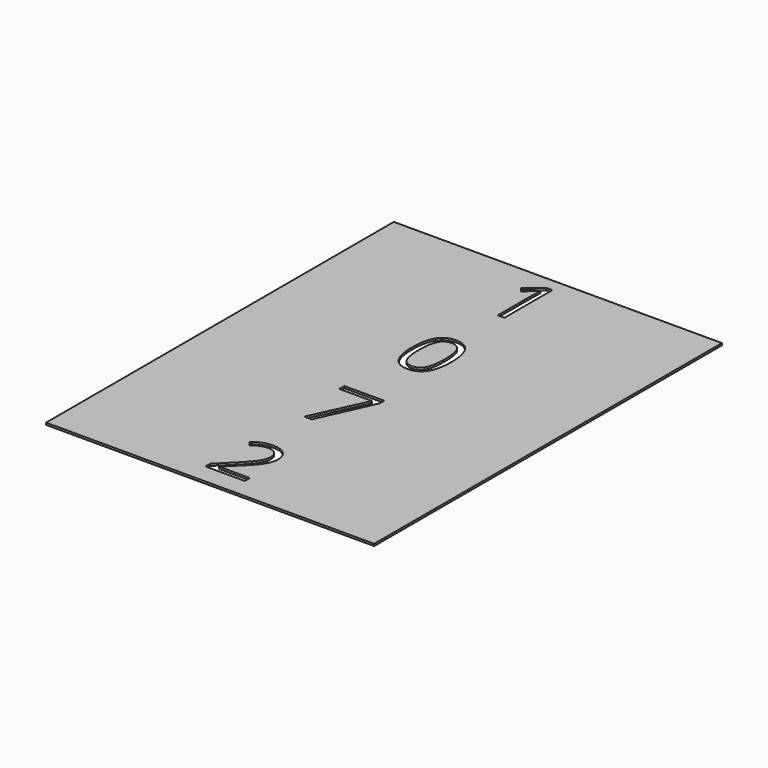
from build123d import *

# Parameters (mm, degrees)
F0_W     = 508
F0_H     = 673.1
F1_DEPTH = 3.175


# Not quite as in the source:
# - a feature names something its author has since deleted; it is built from what else it names


with BuildPart() as f1:
    # F0 (on Top) → F1 (new body)
    with BuildSketch(Plane.XY):
        with Locations((254, -336.55)):
            Rectangle(F0_W, F0_H)
        with BuildLine():
            Line((283.1734824281, -632.5249201278), (283.1734824281, -642.2832268371))
            Line((283.1734824281, -642.2832268371), (222.25, -642.2832268371))
            Line((222.25, -642.2832268371), (222.25, -633.2146964856))
            Line((222.25, -633.2146964856), (246.6559105431, -608.6870607029))
            add(Edge.make_bspline(
                [(246.6559105431, -608.6870607029), (257.814057508, -597.3869009585), (261.3643769968, -592.5686102236)],
                knots=[0, 0, 0, 1, 1, 1], degree=2))
            add(Edge.make_bspline(
                [(261.3643769968, -592.5686102236), (264.9146964856, -587.7503194888), (266.68985623, -583.1856230032)],
                knots=[0, 0, 0, 1, 1, 1], degree=2))
            add(Edge.make_bspline(
                [(266.68985623, -583.1856230032), (268.4650159744, -578.6209265176), (268.4650159744, -573.3664536741)],
                knots=[0, 0, 0, 1, 1, 1], degree=2))
            add(Edge.make_bspline(
                [(268.4650159744, -573.3664536741), (268.4650159744, -565.9412140575), (263.9611821086, -561.5996805112)],
                knots=[0, 0, 0, 1, 1, 1], degree=2))
            add(Edge.make_bspline(
                [(263.9611821086, -561.5996805112), (259.4573482428, -557.2581469649), (251.464057508, -557.2581469649)],
                knots=[0, 0, 0, 1, 1, 1], degree=2))
            add(Edge.make_bspline(
                [(251.464057508, -557.2581469649), (245.7023961661, -557.2581469649), (240.5290734824, -559.1651757189)],
                knots=[0, 0, 0, 1, 1, 1], degree=2))
            add(Edge.make_bspline(
                [(240.5290734824, -559.1651757189), (235.3557507987, -561.0722044728), (229.0260383387, -566.0832268371)],
                knots=[0, 0, 0, 1, 1, 1], degree=2))
            Line((229.0260383387, -566.0832268371), (223.4469648562, -558.9217252396))
            add(Edge.make_bspline(
                [(223.4469648562, -558.9217252396), (236.2484025559, -548.2707667732), (251.3423322684, -548.2707667732)],
                knots=[0, 0, 0, 1, 1, 1], degree=2))
            add(Edge.make_bspline(
                [(251.3423322684, -548.2707667732), (264.4075079872, -548.2707667732), (271.8226038339, -554.9555111821)],
                knots=[0, 0, 0, 1, 1, 1], degree=2))
            add(Edge.make_bspline(
                [(271.8226038339, -554.9555111821), (279.2376996805, -561.6402555911), (279.2376996805, -572.9201277955)],
                knots=[0, 0, 0, 1, 1, 1], degree=2))
            add(Edge.make_bspline(
                [(279.2376996805, -572.9201277955), (279.2376996805, -581.7452076677), (274.2875399361, -590.3674121406)],
                knots=[0, 0, 0, 1, 1, 1], degree=2))
            add(Edge.make_bspline(
                [(274.2875399361, -590.3674121406), (269.3373801917, -598.9896166134), (255.7853035144, -612.1765175719)],
                knots=[0, 0, 0, 1, 1, 1], degree=2))
            Line((255.7853035144, -612.1765175719), (235.4977635783, -632.0177316294))
            Line((235.4977635783, -632.0177316294), (235.4977635783, -632.5249201278))
            Line((235.4977635783, -632.5249201278), (283.1734824281, -632.5249201278))
        make_face(mode=Mode.SUBTRACT)
        Polygon((245.6415335463, -465.7004792332), (233.9761980831, -465.7004792332), (272.3805111821, -382.7041533546), (221.8645367412, -382.7041533546), (221.8645367412, -373.0067092652), (283.538658147, -373.0067092652), (283.538658147, -381.4463258786), align=None, mode=Mode.SUBTRACT)
        with BuildLine():
            add(Edge.make_bspline(
                [(275.8496805112, -207.2067891374), (283.6806709265, -219.4503194888), (283.6806709265, -242.6389776358)],
                knots=[0, 0, 0, 1, 1, 1], degree=2))
            add(Edge.make_bspline(
                [(283.6806709265, -242.6389776358), (283.6806709265, -266.6797124601), (276.1032747604, -278.5377795527)],
                knots=[0, 0, 0, 1, 1, 1], degree=2))
            add(Edge.make_bspline(
                [(276.1032747604, -278.5377795527), (268.5258785942, -290.3958466454), (252.9247603834, -290.3958466454)],
                knots=[0, 0, 0, 1, 1, 1], degree=2))
            add(Edge.make_bspline(
                [(252.9247603834, -290.3958466454), (237.9728434505, -290.3958466454), (230.172284345, -278.2537539936)],
                knots=[0, 0, 0, 1, 1, 1], degree=2))
            add(Edge.make_bspline(
                [(230.172284345, -278.2537539936), (222.3717252396, -266.1116613419), (222.3717252396, -242.6389776358)],
                knots=[0, 0, 0, 1, 1, 1], degree=2))
            add(Edge.make_bspline(
                [(222.3717252396, -242.6389776358), (222.3717252396, -218.435942492), (229.9186900958, -206.699600639)],
                knots=[0, 0, 0, 1, 1, 1], degree=2))
            add(Edge.make_bspline(
                [(229.9186900958, -206.699600639), (237.4656549521, -194.9632587859), (252.9247603834, -194.9632587859)],
                knots=[0, 0, 0, 1, 1, 1], degree=2))
            add(Edge.make_bspline(
                [(252.9247603834, -194.9632587859), (268.0186900958, -194.9632587859), (275.8496805112, -207.2067891374)],
                knots=[0, 0, 0, 1, 1, 1], degree=2))
        make_face(mode=Mode.SUBTRACT)
        with BuildLine():
            Line((261.2223642173, -19.8412140575), (261.2223642173, -112.5349840256))
            Line((261.2223642173, -112.5349840256), (250.9568690096, -112.5349840256))
            Line((250.9568690096, -112.5349840256), (250.9568690096, -46.4787539936))
            add(Edge.make_bspline(
                [(250.9568690096, -46.4787539936), (250.9568690096, -38.2217252396), (251.464057508, -30.8776357827)],
                knots=[0, 0, 0, 1, 1, 1], degree=2))
            add(Edge.make_bspline(
                [(251.464057508, -30.8776357827), (250.1453674121, -32.2166134185), (248.4919329073, -33.667172524)],
                knots=[0, 0, 0, 1, 1, 1], degree=2))
            add(Edge.make_bspline(
                [(248.4919329073, -33.667172524), (246.8384984026, -35.1177316294), (233.4081469649, -46.032428115)],
                knots=[0, 0, 0, 1, 1, 1], degree=2))
            Line((233.4081469649, -46.032428115), (227.8290734824, -38.8100638978))
            Line((227.8290734824, -38.8100638978), (252.3567092652, -19.8412140575))
            Line((252.3567092652, -19.8412140575), (261.2223642173, -19.8412140575))
        make_face(mode=Mode.SUBTRACT)
    extrude(amount=F1_DEPTH)


with BuildPart() as f1b:
    # F0 (on Top) → F1, piece 2 (new body)
    with BuildSketch(Plane.XY):
        with BuildLine():
            add(Edge.make_bspline(
                [(237.7801118211, -213.2524760383), (233.0226837061, -222.4123003195), (233.0226837061, -242.6389776358)],
                knots=[0, 0, 0, 1, 1, 1], degree=2))
            add(Edge.make_bspline(
                [(233.0226837061, -242.6389776358), (233.0226837061, -262.8656549521), (237.7801118211, -272.096485623)],
                knots=[0, 0, 0, 1, 1, 1], degree=2))
            add(Edge.make_bspline(
                [(237.7801118211, -272.096485623), (242.5375399361, -281.3273162939), (252.9247603834, -281.3273162939)],
                knots=[0, 0, 0, 1, 1, 1], degree=2))
            add(Edge.make_bspline(
                [(252.9247603834, -281.3273162939), (263.4539936102, -281.3273162939), (268.1708466454, -271.9747603834)],
                knots=[0, 0, 0, 1, 1, 1], degree=2))
            add(Edge.make_bspline(
                [(268.1708466454, -271.9747603834), (272.8876996805, -262.6222044728), (272.8876996805, -242.6389776358)],
                knots=[0, 0, 0, 1, 1, 1], degree=2))
            add(Edge.make_bspline(
                [(272.8876996805, -242.6389776358), (272.8876996805, -222.6760383387), (268.1708466454, -213.3843450479)],
                knots=[0, 0, 0, 1, 1, 1], degree=2))
            add(Edge.make_bspline(
                [(268.1708466454, -213.3843450479), (263.4539936102, -204.0926517572), (252.9247603834, -204.0926517572)],
                knots=[0, 0, 0, 1, 1, 1], degree=2))
            add(Edge.make_bspline(
                [(252.9247603834, -204.0926517572), (242.5375399361, -204.0926517572), (237.7801118211, -213.2524760383)],
                knots=[0, 0, 0, 1, 1, 1], degree=2))
        make_face()
    extrude(amount=F1_DEPTH)


solid = Compound([f1.part, f1b.part])
